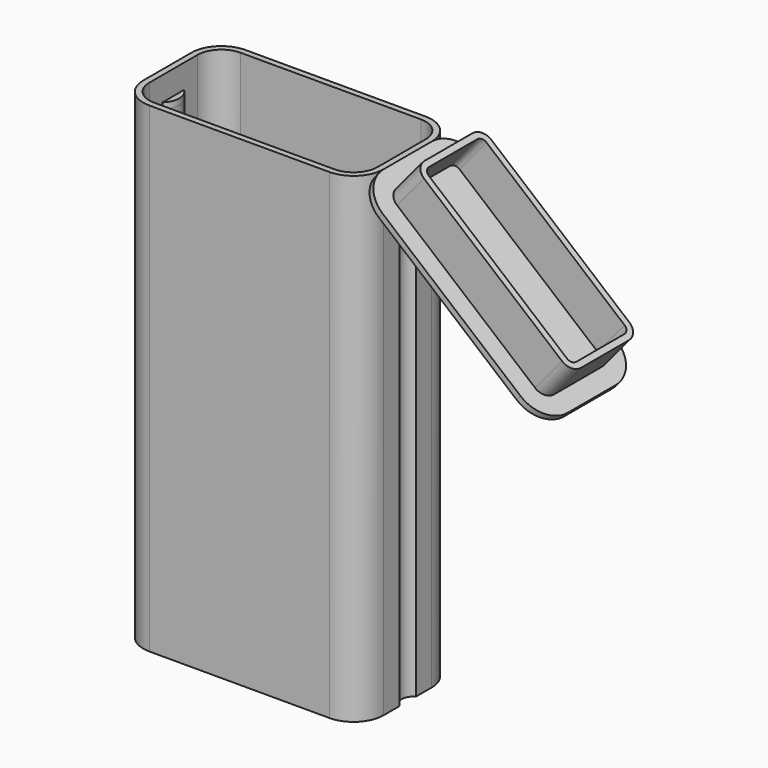
from build123d import *

# Parameters (mm, degrees)
F0_W        = 40
F0_H        = 20
F1_DEPTH    = 80
F2_R        = 5
F4_DEPTH    = 75
F5_T        = 1
F5_T4_ANGLE = 120.000000001
F5_T6_ANGLE = 120.000000001
F7_DEPTH    = 8
F8_ANGLE    = 220
F11_DEPTH   = 7
F12_T       = -1


# Not quite as in the source:
# - a shell that OpenCascade refuses in one call is made with other operations: the cavity is built on its own and cut out


with BuildPart() as f1:
    # F0 (on Top) → F1 (new body)
    with BuildSketch(Plane.XY):
        with Locations((20, 10)):
            Rectangle(F0_W, F0_H)
    extrude(amount=F1_DEPTH)

    # F2
    f2_edges = [f1.edges().sort_by_distance(p)[0] for p in [
        (40, 0, 40),
        (0, 0, 40),
        (40, 20, 40),
        (0, 20, 40),
    ]]
    fillet(f2_edges, radius=F2_R)

    # F3 (on face) → F4 (cut)
    with BuildSketch(Plane(origin=(0, 0, 0), x_dir=(1, 0, 0), z_dir=(0, 0, -1))):
        with BuildLine():
            Line((0, -8.2679491924), (0, -11.7320508076))
            ThreePointArc((0, -11.7320508076), (1, -10), (0, -8.2679491924))
        make_face()
        with BuildLine():
            ThreePointArc((40, -8.2679491924), (39, -10), (40, -11.7320508076))
            Line((40, -11.7320508076), (40, -8.2679491924))
        make_face()
    extrude(amount=-F4_DEPTH, mode=Mode.SUBTRACT)

    # F5: shell of thickness 1, made by hand


with BuildPart() as f5_core1:
    # F5_t2: copy of F1
    add(f1.part)

    # the walls: a layer under each face that stays
    f5_faces = [f5_core1.faces().sort_by_distance(p)[0] for p in [
        (0, 13.3333333333, 66.6666666667),
        (20, 10, 0),
        (1, 10, 37.5),
        (0.5, 10, 75),
        (1.4644660941, 1.4644660941, 40),
        (1.4644660941, 18.5355339059, 40),
        (20, 20, 40),
        (38.5355339059, 18.5355339059, 40),
        (40, 6.6666666667, 66.6666666667),
        (39, 10, 37.5),
        (38.5355339059, 1.4644660941, 40),
        (20, 0, 40),
        (39.5, 10, 75),
    ]]
    thicken(f5_faces, amount=-F5_T, mode=Mode.SUBTRACT)

    # F5_s3 → F5_t4 (revolve, cut)
    with BuildSketch(Plane(origin=(-5.0801270189, 2.9330127019, 0), x_dir=(0, 0, 1), z_dir=(-0.8660254038, 0.5, 0))):
        Polygon((74.99, 10.1502540378), (75, 11.1602540378), (76, 11.1602540378), (76, 10.1602540378), align=None)
    revolve(axis=Axis((-1, 10, 75), (0, 0, -1)), revolution_arc=F5_T4_ANGLE, mode=Mode.SUBTRACT)

    # F5_s5 → F5_t6 (revolve, cut)
    with BuildSketch(Plane(origin=(26.4198729811, -15.2535207776, 0), x_dir=(0, 0, 1), z_dir=(0.8660254038, -0.5, 0))):
        Polygon((74.99, -27.1702540378), (75, -26.1602540378), (76, -26.1602540378), (76, -27.1602540378), align=None)
    revolve(axis=Axis((41, 10, 75), (0, 0, -1)), revolution_arc=F5_T6_ANGLE, mode=Mode.SUBTRACT)


with BuildPart() as f1_1:
    add(f1.part)

    # what is left inside the walls is the cavity
    f5_cavity = [f5_core1.part.solids().sort_by_distance(p)[0] for p in [
        (20, 1.01, 53.666667),
    ]]
    add(f5_cavity, mode=Mode.SUBTRACT)


with BuildPart() as f7:
    # F6 (on face) → F7 (new body)
    with BuildSketch(Plane.XY.offset(80)):
        with BuildLine():
            ThreePointArc((35, 0), (38.5355339059, 1.4644660941), (40, 5))
            Line((40, 5), (40, 15))
            ThreePointArc((40, 15), (38.5355339059, 18.5355339059), (35, 20))
            Line((35, 20), (5, 20))
            ThreePointArc((5, 20), (1.4644660941, 18.5355339059), (0, 15))
            Line((0, 15), (0, 5))
            ThreePointArc((0, 5), (1.4644660941, 1.4644660941), (5, 0))
            Line((5, 0), (35, 0))
        make_face()
    extrude(amount=F7_DEPTH)


with BuildPart() as f7_1:
    # F8: moved
    add(f7.part.rotate(Axis((40, 10, 80), (0, 1, 0)), F8_ANGLE))


with BuildPart() as f7_2:
    # F9: moved
    add(f7_1.part.moved(Location((4.4995132678, 0, 5.3623111018))))

    # F10 (on face) → F11 (cut)
    with BuildSketch(Plane(origin=(60.418859835, 0, 72.0043932688), x_dir=(0.7660444431, 0, -0.6427876097), z_dir=(0.6427876097, 0, 0.7660444431))):
        with BuildLine():
            ThreePointArc((19.2187689498, 15), (17.7543028558, 18.5355339059), (14.2187689498, 20))
            Line((14.2187689498, 20), (-15.7812310502, 20))
            ThreePointArc((-15.7812310502, 20), (-19.3167649561, 18.5355339059), (-20.7812310502, 15))
            Line((-20.7812310502, 15), (-20.7812310502, 5))
            ThreePointArc((-20.7812310502, 5), (-19.3167649561, 1.4644660941), (-15.7812310502, 0))
            Line((-15.7812310502, 0), (14.2187689498, 0))
            ThreePointArc((14.2187689498, 0), (17.7543028558, 1.4644660941), (19.2187689498, 5))
            Line((19.2187689498, 5), (19.2187689498, 15))
        make_face()
        with BuildLine():
            ThreePointArc((14.2187689498, 17.0000009239), (15.6329831655, 16.4142142156), (16.2187698737, 15))
            Line((16.2187698737, 15), (16.2187698737, 5))
            ThreePointArc((16.2187698737, 5), (15.6329831655, 3.5857857844), (14.2187689498, 2.9999990761))
            Line((14.2187689498, 2.9999990761), (-15.7812310502, 2.9999990761))
            ThreePointArc((-15.7812310502, 2.9999990761), (-17.1954452658, 3.5857857844), (-17.781231974, 5))
            Line((-17.781231974, 5), (-17.781231974, 15))
            ThreePointArc((-17.781231974, 15), (-17.1954452658, 16.4142142156), (-15.7812310502, 17.0000009239))
            Line((-15.7812310502, 17.0000009239), (14.2187689498, 17.0000009239))
        make_face(mode=Mode.SUBTRACT)
    extrude(amount=-F11_DEPTH, mode=Mode.SUBTRACT)

    # F12
    f12_openings = [f7_2.faces().sort_by_distance(p)[0] for p in [
        (59.820402, 10, 72.506559),
    ]]
    offset(amount=F12_T, openings=f12_openings, kind=Kind.INTERSECTION)


solid = Compound([f1_1.part, f7_2.part])
